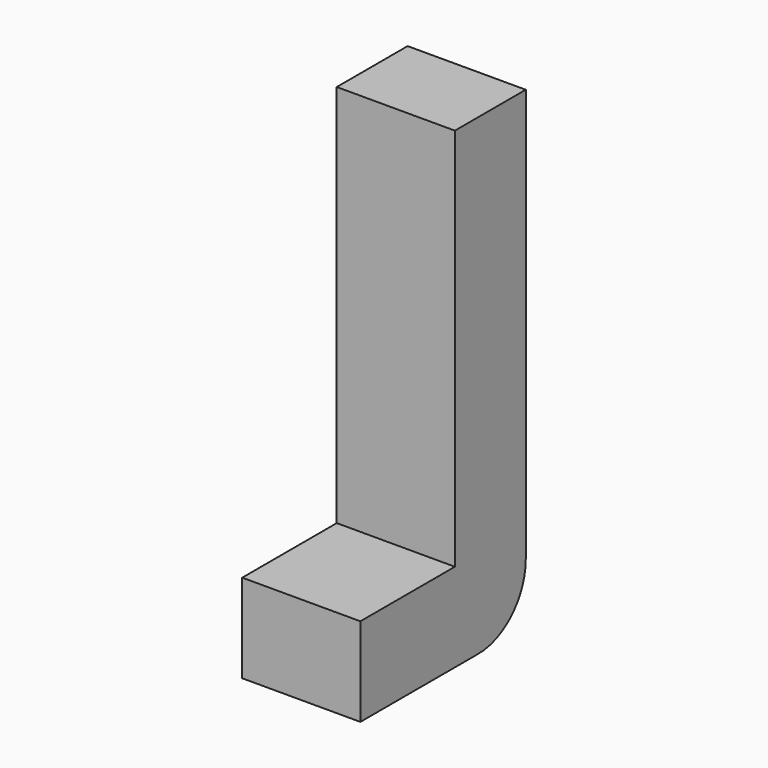
from build123d import *

# Parameters (mm, degrees)
F0_W     = 76.2
F0_H     = 330.2
F1_DEPTH = 101.6


# Not quite as in the source:
# - a feature of the source that left no trace in its solid (it failed there, or was rolled back) is left out


with BuildPart() as f1:
    # F0 (on Right) → F1 (new body)
    with BuildSketch(Plane.YZ):
        with Locations((-103.380974756, -25.9231243968)):
            Rectangle(F0_W, F0_H)
        with BuildLine():
            Line((-65.280974756, -191.0231243968), (-141.480974756, -191.0231243968))
            Line((-141.480974756, -191.0231243968), (-243.080974756, -191.0231243968))
            Line((-243.080974756, -191.0231243968), (-243.080974756, -267.2231243968))
            Line((-243.080974756, -267.2231243968), (-116.080974756, -267.2231243968))
            ThreePointArc((-116.080974756, -267.2231243968), (-80.1599502717, -252.3441488811), (-65.280974756, -216.4231243968))
            Line((-65.280974756, -216.4231243968), (-65.280974756, -191.0231243968))
        make_face()
    extrude(amount=F1_DEPTH)


solid = f1.part
